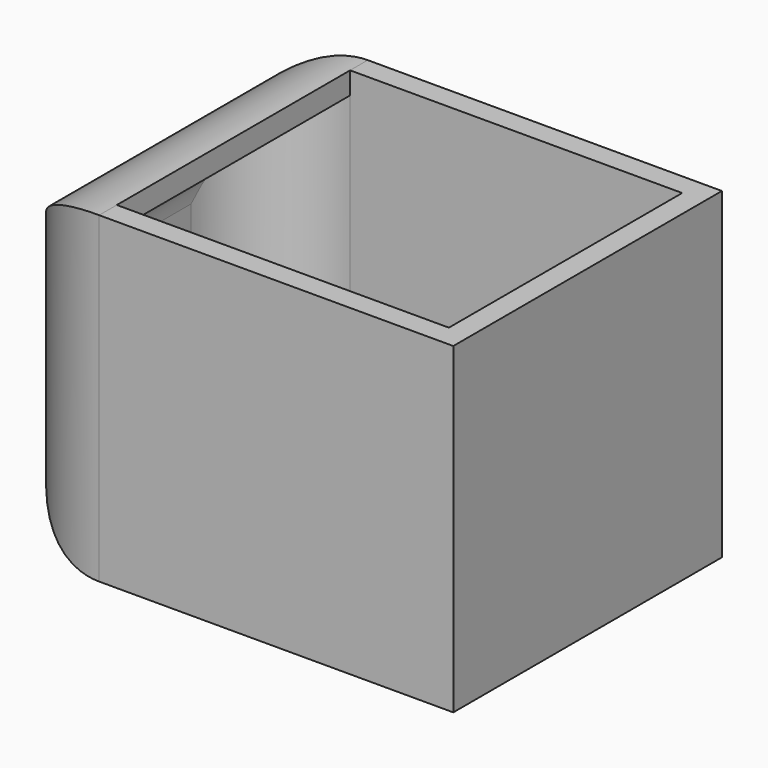
from build123d import *

# Parameters (mm, degrees)
F0_W     = 53.4262955189
F0_H     = 38.6142134666
F1_DEPTH = 37.0909944177
F2_R     = 12.7
F3_T     = -2.54


# Not quite as in the source:
# - a shell that OpenCascade refuses in one call is made with other operations: the cavity is built on its own and cut out


with BuildPart() as f1:
    # F0 (on Top) → F1 (new body)
    with BuildSketch(Plane.XY):
        with Locations((-26.7131477594, 19.3071067333)):
            Rectangle(F0_W, F0_H)
    extrude(amount=F1_DEPTH)

    # F2
    f2_edges = [f1.edges().sort_by_distance(p)[0] for p in [
        (-53.426296, 38.614213, 18.545497),
        (-53.426296, 0, 18.545497),
        (-53.426296, 19.307107, 0),
        (-53.426296, 19.307107, 37.090994),
    ]]
    fillet(f2_edges, radius=F2_R)

    # F3: a shell. OpenCascade refuses it in one call, so the cavity is built on its own and cut out:
    # the body offset inwards by the wall thickness, plus a prism from it out through each open face.
    f3_core = offset(f1.part, amount=F3_T, mode=Mode.PRIVATE)
    f3_exits = [f3_core.faces().sort_by_distance(p)[0] for p in [
        (-21.633148, 19.307107, 34.550994),
    ]]
    add(f3_core, mode=Mode.SUBTRACT)
    extrude(f3_exits, amount=-F3_T, mode=Mode.SUBTRACT)


solid = f1.part
